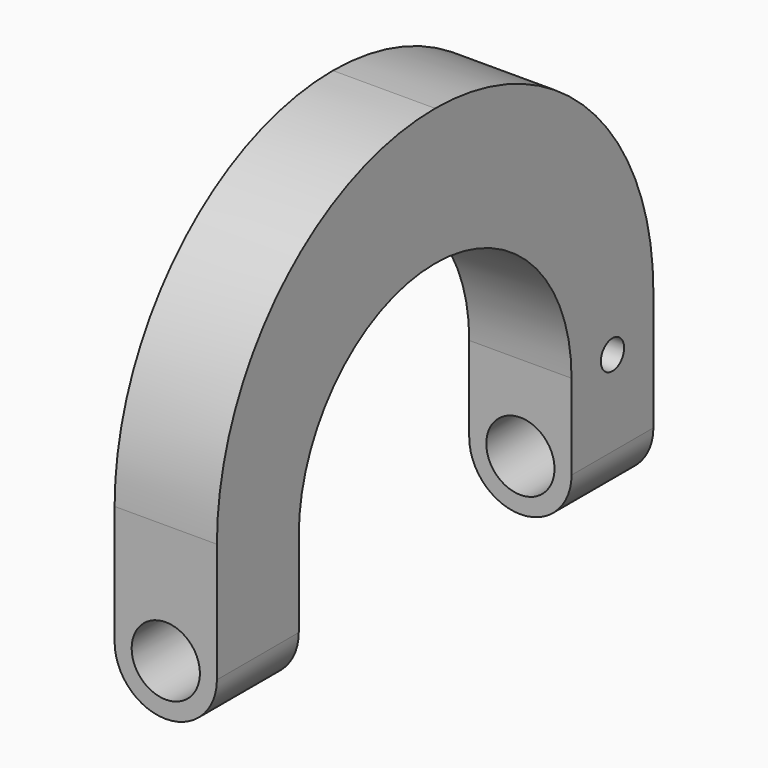
from build123d import *

# Parameters (mm, degrees)
F0_R     = 1.35255
F1_DEPTH = 9.525
F2_R     = 3.175
F3_DEPTH = 50.8
F4_R     = 1.190625
F5_DEPTH = 6.35


# Not quite as in the source:
# - a feature names something its author has since deleted; it is built from what else it names


with BuildPart() as f1:
    # F0 (on Right) → F1 (new body)
    with BuildSketch(Plane.YZ):
        with BuildLine():
            Line((-15.875, -12.7), (-15.875, 0))
            ThreePointArc((-15.875, 0), (-11.2253201513, 11.2253201513), (0, 15.875))
            ThreePointArc((0, 15.875), (11.2253201513, 11.2253201513), (15.875, 0))
            Line((15.875, 0), (15.875, -12.7))
            Line((15.875, -12.7), (25.4, -12.7))
            Line((25.4, -12.7), (25.4, 0))
            Line((25.4, 0), (25.4, 3.175))
            ThreePointArc((25.4, 3.175), (17.9605122421, 21.1355122421), (0, 28.575))
            ThreePointArc((0, 28.575), (-17.9605122421, 21.1355122421), (-25.4, 3.175))
            Line((-25.4, 3.175), (-25.4, 0))
            Line((-25.4, 0), (-25.4, -12.7))
            Line((-25.4, -12.7), (-15.875, -12.7))
        make_face()
        with Locations((20.6375, 0)):
            Circle(F0_R, mode=Mode.SUBTRACT)
    extrude(amount=F1_DEPTH)

    # F2 (on face) → F3 (cut)
    with BuildSketch(Plane(origin=(0, 25.4, 0), x_dir=(-1, 0, 0), z_dir=(0, 1, 0))):
        with Locations((-4.7625, -7.9375)):
            Circle(F2_R)
        with BuildLine():
            ThreePointArc((-4.7625, -12.7), (-8.1300960454, -11.3050960454), (-9.525, -7.9375))
            Line((-9.525, -7.9375), (-9.525, -12.7))
            Line((-9.525, -12.7), (-4.7625, -12.7))
        make_face()
        with BuildLine():
            ThreePointArc((0, -7.9375), (-1.3949039546, -11.3050960454), (-4.7625, -12.7))
            Line((-4.7625, -12.7), (0, -12.7))
            Line((0, -12.7), (0, -7.9375))
        make_face()
    extrude(amount=-F3_DEPTH, mode=Mode.SUBTRACT)

    # F4 (on Top) → F5 (cut)
    with BuildSketch(Plane.XY):
        with Locations((4.7625, -19.05)):
            Circle(F4_R)
    extrude(amount=-F5_DEPTH, mode=Mode.SUBTRACT)


solid = f1.part
